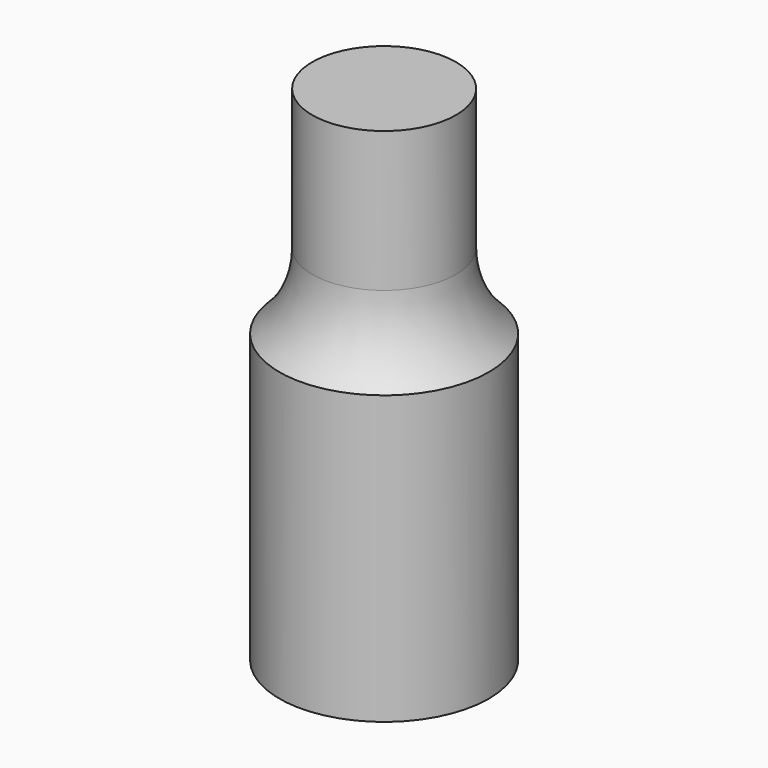
from build123d import *


# Not quite as in the source:
# - a fillet or chamfer that OpenCascade refuses, or shapes differently, is made with other operations: its cross-section is extruded or revolved along the edge and cut away or added


with BuildPart() as f1:
    # F0 (on Front) → F1 (revolve)
    with BuildSketch(Plane.XZ):
        Polygon((4.1, -14), (5.1, -14), (5.1, 0), (3.5, 0), (3.5, 10.5), (0, 10.5), (0, 10), (2.7, 10), (2.7, -2), (4.1, -2), align=None)
    revolve(axis=Axis((0, 0, -6.7832856439), (0, 0, -1)))

    # F2: fillet of radius 5 on 1 edges, made by hand

    # F2_s1 → F2_t2 (revolve)
    with BuildSketch(Plane.XZ):
        with BuildLine():
            ThreePointArc((5.1, 0), (3.917424305, 1.666060556), (3.5, 3.666060556))
            Line((3.5, 3.666060556), (3.5, 0))
            Line((3.5, 0), (5.1, 0))
        make_face()
    revolve(axis=Axis((0, 0, 0), (0, 0, -1)))


solid = f1.part
